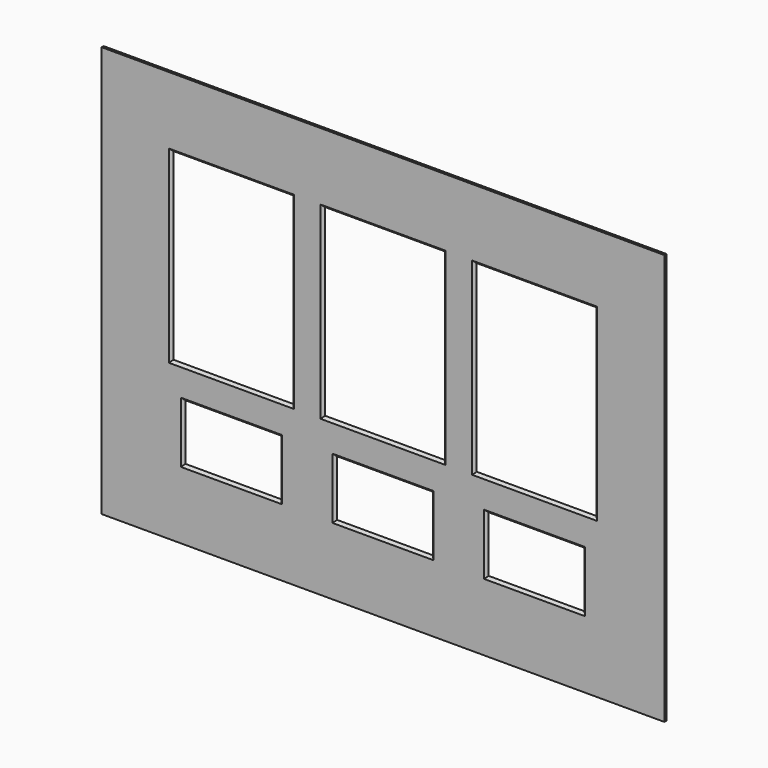
from build123d import *

# Parameters (mm, degrees)
F0_W          = 447.675
F0_H          = 327.025
F0_W_2        = 76.2
F0_H_2        = 44.45
F0_W_3        = 95.25
F0_H_3        = 146.05
F1_DEPTH      = 2
F2_T1_DEPTH   = 95.25
F2_T3_DEPTH   = 146.05
F2_T5_DEPTH   = 95.25
F2_T7_DEPTH   = 95.25
F2_T9_DEPTH   = 76.2
F2_T11_DEPTH  = 44.45
F2_T13_DEPTH  = 76.2
F2_T15_DEPTH  = 76.2
F2_T21_DEPTH  = 151.2756598315
F2_T25_DEPTH  = 100.4756598315
F2_T32_DEPTH  = 100.4756598315
F2_T36_DEPTH  = 151.2756598315
F2_T43_DEPTH  = 151.2756598315
F2_T47_DEPTH  = 100.4756598315
F2_T54_DEPTH  = 151.2756598315
F2_T58_DEPTH  = 100.4756598315
F2_T65_DEPTH  = 151.2756598315
F2_T69_DEPTH  = 100.4756598315
F2_T76_DEPTH  = 151.2756598315
F2_T80_DEPTH  = 100.4756598315
F2_T87_DEPTH  = 100.4756598315
F2_T91_DEPTH  = 151.2756598315
F2_T98_DEPTH  = 151.2756598315
F2_T102_DEPTH = 100.4756598315
F2_T109_DEPTH = 151.2756598315
F2_T113_DEPTH = 100.4756598315
F2_T120_DEPTH = 100.4756598315
F2_T124_DEPTH = 151.2756598315
F2_T131_DEPTH = 151.2756598315
F2_T135_DEPTH = 100.4756598315
F2_T142_DEPTH = 151.2756598315
F2_T146_DEPTH = 100.4756598315
F2_T153_DEPTH = 49.6756598315
F2_T157_DEPTH = 81.4256598315
F2_T164_DEPTH = 81.4256598315
F2_T168_DEPTH = 49.6756598315
F2_T175_DEPTH = 49.6756598315
F2_T179_DEPTH = 81.4256598315
F2_T186_DEPTH = 49.6756598315
F2_T190_DEPTH = 81.4256598315
F2_T197_DEPTH = 81.4256598315
F2_T201_DEPTH = 49.6756598315
F2_T208_DEPTH = 81.4256598315
F2_T212_DEPTH = 49.6756598315
F2_T219_DEPTH = 49.6756598315
F2_T223_DEPTH = 81.4256598315
F2_T230_DEPTH = 81.4256598315
F2_T234_DEPTH = 49.6756598315
F2_T241_DEPTH = 49.6756598315
F2_T245_DEPTH = 81.4256598315
F2_T252_DEPTH = 81.4256598315
F2_T256_DEPTH = 49.6756598315
F2_T263_DEPTH = 81.4256598315
F2_T267_DEPTH = 49.6756598315
F2_T274_DEPTH = 81.4256598315
F2_T278_DEPTH = 49.6756598315


# Not quite as in the source:
# - a fillet or chamfer that OpenCascade refuses, or shapes differently, is made with other operations: its cross-section is extruded or revolved along the edge and cut away or added


with BuildPart() as f1:
    # F0 (on Front) → F1 (new body)
    with BuildSketch(Plane.XZ):
        Rectangle(F0_W, F0_H)
        with Locations((-120.65, -85.725)):
            Rectangle(F0_W_2, F0_H_2, mode=Mode.SUBTRACT)
        with Locations((0, -85.725)):
            Rectangle(F0_W_2, F0_H_2, mode=Mode.SUBTRACT)
        with Locations((120.65, -85.725)):
            Rectangle(F0_W_2, F0_H_2, mode=Mode.SUBTRACT)
        with Locations((-120.65, 34.925)):
            Rectangle(F0_W_3, F0_H_3, mode=Mode.SUBTRACT)
        with Locations((0, 34.925)):
            Rectangle(F0_W_3, F0_H_3, mode=Mode.SUBTRACT)
        with Locations((120.65, 34.925)):
            Rectangle(F0_W_3, F0_H_3, mode=Mode.SUBTRACT)
    extrude(amount=F1_DEPTH)

    # F2: chamfer of 2.032 on 24 edges, made by hand

    # F2_s2 → F2_t1 (cut)
    with BuildSketch(Plane.YZ.offset(-168.275)):
        Polygon((0.032, 107.95), (-2, 109.982), (-2, 107.95), align=None)
        Polygon((0.032, -38.1), (-2, -40.132), (-2, -38.1), align=None)
    extrude(amount=F2_T1_DEPTH, mode=Mode.SUBTRACT)

    # F2_s4 → F2_t3 (cut)
    with BuildSketch(Plane.XY.offset(-38.1)):
        Polygon((-168.275, 0.032), (-170.307, -2), (-168.275, -2), align=None)
        Polygon((-73.025, 0.032), (-70.993, -2), (-73.025, -2), align=None)
        Polygon((-47.625, 0.032), (-49.657, -2), (-47.625, -2), align=None)
        Polygon((47.625, 0.032), (49.657, -2), (47.625, -2), align=None)
        Polygon((73.025, 0.032), (70.993, -2), (73.025, -2), align=None)
        Polygon((168.275, 0.032), (170.307, -2), (168.275, -2), align=None)
    extrude(amount=F2_T3_DEPTH, mode=Mode.SUBTRACT)

    # F2_s6 → F2_t5 (cut)
    with BuildSketch(Plane.YZ.offset(-47.625)):
        Polygon((0.032, 107.95), (-2, 109.982), (-2, 107.95), align=None)
        Polygon((0.032, -38.1), (-2, -40.132), (-2, -38.1), align=None)
    extrude(amount=F2_T5_DEPTH, mode=Mode.SUBTRACT)

    # F2_s8 → F2_t7 (cut)
    with BuildSketch(Plane.YZ.offset(73.025)):
        Polygon((0.032, -38.1), (-2, -40.132), (-2, -38.1), align=None)
        Polygon((0.032, 107.95), (-2, 109.982), (-2, 107.95), align=None)
    extrude(amount=F2_T7_DEPTH, mode=Mode.SUBTRACT)

    # F2_s10 → F2_t9 (cut)
    with BuildSketch(Plane.YZ.offset(82.55)):
        Polygon((0.032, -63.5), (-2, -61.468), (-2, -63.5), align=None)
        Polygon((0.032, -107.95), (-2, -109.982), (-2, -107.95), align=None)
    extrude(amount=F2_T9_DEPTH, mode=Mode.SUBTRACT)

    # F2_s12 → F2_t11 (cut)
    with BuildSketch(Plane.XY.offset(-107.95)):
        Polygon((158.75, 0.032), (160.782, -2), (158.75, -2), align=None)
        Polygon((82.55, 0.032), (80.518, -2), (82.55, -2), align=None)
        Polygon((38.1, 0.032), (40.132, -2), (38.1, -2), align=None)
        Polygon((-38.1, 0.032), (-40.132, -2), (-38.1, -2), align=None)
        Polygon((-82.55, 0.032), (-80.518, -2), (-82.55, -2), align=None)
        Polygon((-158.75, 0.032), (-160.782, -2), (-158.75, -2), align=None)
    extrude(amount=F2_T11_DEPTH, mode=Mode.SUBTRACT)

    # F2_s14 → F2_t13 (cut)
    with BuildSketch(Plane.YZ.offset(-38.1)):
        Polygon((0.032, -63.5), (-2, -61.468), (-2, -63.5), align=None)
        Polygon((0.032, -107.95), (-2, -109.982), (-2, -107.95), align=None)
    extrude(amount=F2_T13_DEPTH, mode=Mode.SUBTRACT)

    # F2_s16 → F2_t15 (cut)
    with BuildSketch(Plane.YZ.offset(-158.75)):
        Polygon((0.032, -107.95), (-2, -109.982), (-2, -107.95), align=None)
        Polygon((0.032, -63.5), (-2, -61.468), (-2, -63.5), align=None)
    extrude(amount=F2_T15_DEPTH, mode=Mode.SUBTRACT)


with BuildPart() as f2_tool19:
    # F2_s20 → F2_t21 (new body)
    with BuildSketch(Plane.XY.offset(-38.1)):
        Polygon((-168.275, 0.032), (-170.307, -2), (-168.275, -2), align=None)
    extrude(amount=F2_T21_DEPTH)

    split(bisect_by=Plane.XY.offset(107.95), keep=Keep.TOP)


with BuildPart() as f2_tool23:
    # F2_s24 → F2_t25 (new body)
    with BuildSketch(Plane.YZ.offset(-173.5006598315)):
        Polygon((0.032, 107.95), (-2, 109.982), (-2, 107.95), align=None)
    extrude(amount=F2_T25_DEPTH)

    split(bisect_by=Plane.YZ.offset(-168.275), keep=Keep.BOTTOM)


with BuildPart() as f2_tool19_1:
    add(f2_tool19.part)

    # F2_t27: intersect F2_tool23
    add(f2_tool23.part, mode=Mode.INTERSECT)


with BuildPart() as f1_1:
    add(f1.part)

    # F2_t17: cut F2_tool19
    add(f2_tool19_1.part, mode=Mode.SUBTRACT)


with BuildPart() as f2_tool30:
    # F2_s31 → F2_t32 (new body)
    with BuildSketch(Plane.YZ.offset(-168.275)):
        Polygon((0.032, 107.95), (-2, 109.982), (-2, 107.95), align=None)
    extrude(amount=F2_T32_DEPTH)

    split(bisect_by=Plane.YZ.offset(-73.025), keep=Keep.TOP)


with BuildPart() as f2_tool34:
    # F2_s35 → F2_t36 (new body)
    with BuildSketch(Plane.XY.offset(113.1756598315)):
        Polygon((-73.025, 0.032), (-70.993, -2), (-73.025, -2), align=None)
    extrude(amount=-F2_T36_DEPTH)

    split(bisect_by=Plane.XY.offset(107.95), keep=Keep.TOP)


with BuildPart() as f2_tool30_1:
    add(f2_tool30.part)

    # F2_t38: intersect F2_tool34
    add(f2_tool34.part, mode=Mode.INTERSECT)


with BuildPart() as f1_2:
    add(f1_1.part)

    # F2_t28: cut F2_tool30
    add(f2_tool30_1.part, mode=Mode.SUBTRACT)


with BuildPart() as f2_tool41:
    # F2_s42 → F2_t43 (new body)
    with BuildSketch(Plane.XY.offset(-43.3256598315)):
        Polygon((-168.275, 0.032), (-170.307, -2), (-168.275, -2), align=None)
    extrude(amount=F2_T43_DEPTH)

    split(bisect_by=Plane.XY.offset(-38.1), keep=Keep.BOTTOM)


with BuildPart() as f2_tool45:
    # F2_s46 → F2_t47 (new body)
    with BuildSketch(Plane.YZ.offset(-73.025)):
        Polygon((0.032, -38.1), (-2, -40.132), (-2, -38.1), align=None)
    extrude(amount=-F2_T47_DEPTH)

    split(bisect_by=Plane.YZ.offset(-168.275), keep=Keep.BOTTOM)


with BuildPart() as f2_tool41_1:
    add(f2_tool41.part)

    # F2_t49: intersect F2_tool45
    add(f2_tool45.part, mode=Mode.INTERSECT)


with BuildPart() as f1_3:
    add(f1_2.part)

    # F2_t39: cut F2_tool41
    add(f2_tool41_1.part, mode=Mode.SUBTRACT)


with BuildPart() as f2_tool52:
    # F2_s53 → F2_t54 (new body)
    with BuildSketch(Plane.XY.offset(107.95)):
        Polygon((-73.025, 0.032), (-70.993, -2), (-73.025, -2), align=None)
    extrude(amount=-F2_T54_DEPTH)

    split(bisect_by=Plane.XY.offset(-38.1), keep=Keep.BOTTOM)


with BuildPart() as f2_tool56:
    # F2_s57 → F2_t58 (new body)
    with BuildSketch(Plane.YZ.offset(-67.7993401685)):
        Polygon((0.032, -38.1), (-2, -40.132), (-2, -38.1), align=None)
    extrude(amount=-F2_T58_DEPTH)

    split(bisect_by=Plane.YZ.offset(-73.025), keep=Keep.TOP)


with BuildPart() as f2_tool52_1:
    add(f2_tool52.part)

    # F2_t60: intersect F2_tool56
    add(f2_tool56.part, mode=Mode.INTERSECT)


with BuildPart() as f1_4:
    add(f1_3.part)

    # F2_t50: cut F2_tool52
    add(f2_tool52_1.part, mode=Mode.SUBTRACT)


with BuildPart() as f2_tool63:
    # F2_s64 → F2_t65 (new body)
    with BuildSketch(Plane.XY.offset(-38.1)):
        Polygon((-47.625, 0.032), (-49.657, -2), (-47.625, -2), align=None)
    extrude(amount=F2_T65_DEPTH)

    split(bisect_by=Plane.XY.offset(107.95), keep=Keep.TOP)


with BuildPart() as f2_tool67:
    # F2_s68 → F2_t69 (new body)
    with BuildSketch(Plane.YZ.offset(-52.8506598315)):
        Polygon((0.032, 107.95), (-2, 109.982), (-2, 107.95), align=None)
    extrude(amount=F2_T69_DEPTH)

    split(bisect_by=Plane.YZ.offset(-47.625), keep=Keep.BOTTOM)


with BuildPart() as f2_tool63_1:
    add(f2_tool63.part)

    # F2_t71: intersect F2_tool67
    add(f2_tool67.part, mode=Mode.INTERSECT)


with BuildPart() as f1_5:
    add(f1_4.part)

    # F2_t61: cut F2_tool63
    add(f2_tool63_1.part, mode=Mode.SUBTRACT)


with BuildPart() as f2_tool74:
    # F2_s75 → F2_t76 (new body)
    with BuildSketch(Plane.XY.offset(113.1756598315)):
        Polygon((47.625, 0.032), (49.657, -2), (47.625, -2), align=None)
    extrude(amount=-F2_T76_DEPTH)

    split(bisect_by=Plane.XY.offset(107.95), keep=Keep.TOP)


with BuildPart() as f2_tool78:
    # F2_s79 → F2_t80 (new body)
    with BuildSketch(Plane.YZ.offset(-47.625)):
        Polygon((0.032, 107.95), (-2, 109.982), (-2, 107.95), align=None)
    extrude(amount=F2_T80_DEPTH)

    split(bisect_by=Plane.YZ.offset(47.625), keep=Keep.TOP)


with BuildPart() as f2_tool74_1:
    add(f2_tool74.part)

    # F2_t82: intersect F2_tool78
    add(f2_tool78.part, mode=Mode.INTERSECT)


with BuildPart() as f1_6:
    add(f1_5.part)

    # F2_t72: cut F2_tool74
    add(f2_tool74_1.part, mode=Mode.SUBTRACT)


with BuildPart() as f2_tool85:
    # F2_s86 → F2_t87 (new body)
    with BuildSketch(Plane.YZ.offset(47.625)):
        Polygon((0.032, -38.1), (-2, -40.132), (-2, -38.1), align=None)
    extrude(amount=-F2_T87_DEPTH)

    split(bisect_by=Plane.YZ.offset(-47.625), keep=Keep.BOTTOM)


with BuildPart() as f2_tool89:
    # F2_s90 → F2_t91 (new body)
    with BuildSketch(Plane.XY.offset(-43.3256598315)):
        Polygon((-47.625, 0.032), (-49.657, -2), (-47.625, -2), align=None)
    extrude(amount=F2_T91_DEPTH)

    split(bisect_by=Plane.XY.offset(-38.1), keep=Keep.BOTTOM)


with BuildPart() as f2_tool85_1:
    add(f2_tool85.part)

    # F2_t93: intersect F2_tool89
    add(f2_tool89.part, mode=Mode.INTERSECT)


with BuildPart() as f1_7:
    add(f1_6.part)

    # F2_t83: cut F2_tool85
    add(f2_tool85_1.part, mode=Mode.SUBTRACT)


with BuildPart() as f2_tool96:
    # F2_s97 → F2_t98 (new body)
    with BuildSketch(Plane.XY.offset(107.95)):
        Polygon((47.625, 0.032), (49.657, -2), (47.625, -2), align=None)
    extrude(amount=-F2_T98_DEPTH)

    split(bisect_by=Plane.XY.offset(-38.1), keep=Keep.BOTTOM)


with BuildPart() as f2_tool100:
    # F2_s101 → F2_t102 (new body)
    with BuildSketch(Plane.YZ.offset(52.8506598315)):
        Polygon((0.032, -38.1), (-2, -40.132), (-2, -38.1), align=None)
    extrude(amount=-F2_T102_DEPTH)

    split(bisect_by=Plane.YZ.offset(47.625), keep=Keep.TOP)


with BuildPart() as f2_tool96_1:
    add(f2_tool96.part)

    # F2_t104: intersect F2_tool100
    add(f2_tool100.part, mode=Mode.INTERSECT)


with BuildPart() as f1_8:
    add(f1_7.part)

    # F2_t94: cut F2_tool96
    add(f2_tool96_1.part, mode=Mode.SUBTRACT)


with BuildPart() as f2_tool107:
    # F2_s108 → F2_t109 (new body)
    with BuildSketch(Plane.XY.offset(107.95)):
        Polygon((168.275, 0.032), (170.307, -2), (168.275, -2), align=None)
    extrude(amount=-F2_T109_DEPTH)

    split(bisect_by=Plane.XY.offset(-38.1), keep=Keep.BOTTOM)


with BuildPart() as f2_tool111:
    # F2_s112 → F2_t113 (new body)
    with BuildSketch(Plane.YZ.offset(173.5006598315)):
        Polygon((0.032, -38.1), (-2, -40.132), (-2, -38.1), align=None)
    extrude(amount=-F2_T113_DEPTH)

    split(bisect_by=Plane.YZ.offset(168.275), keep=Keep.TOP)


with BuildPart() as f2_tool107_1:
    add(f2_tool107.part)

    # F2_t115: intersect F2_tool111
    add(f2_tool111.part, mode=Mode.INTERSECT)


with BuildPart() as f1_9:
    add(f1_8.part)

    # F2_t105: cut F2_tool107
    add(f2_tool107_1.part, mode=Mode.SUBTRACT)


with BuildPart() as f2_tool118:
    # F2_s119 → F2_t120 (new body)
    with BuildSketch(Plane.YZ.offset(168.275)):
        Polygon((0.032, -38.1), (-2, -40.132), (-2, -38.1), align=None)
    extrude(amount=-F2_T120_DEPTH)

    split(bisect_by=Plane.YZ.offset(73.025), keep=Keep.BOTTOM)


with BuildPart() as f2_tool122:
    # F2_s123 → F2_t124 (new body)
    with BuildSketch(Plane.XY.offset(-43.3256598315)):
        Polygon((73.025, 0.032), (70.993, -2), (73.025, -2), align=None)
    extrude(amount=F2_T124_DEPTH)

    split(bisect_by=Plane.XY.offset(-38.1), keep=Keep.BOTTOM)


with BuildPart() as f2_tool118_1:
    add(f2_tool118.part)

    # F2_t126: intersect F2_tool122
    add(f2_tool122.part, mode=Mode.INTERSECT)


with BuildPart() as f1_10:
    add(f1_9.part)

    # F2_t116: cut F2_tool118
    add(f2_tool118_1.part, mode=Mode.SUBTRACT)


with BuildPart() as f2_tool129:
    # F2_s130 → F2_t131 (new body)
    with BuildSketch(Plane.XY.offset(-38.1)):
        Polygon((73.025, 0.032), (70.993, -2), (73.025, -2), align=None)
    extrude(amount=F2_T131_DEPTH)

    split(bisect_by=Plane.XY.offset(107.95), keep=Keep.TOP)


with BuildPart() as f2_tool133:
    # F2_s134 → F2_t135 (new body)
    with BuildSketch(Plane.YZ.offset(67.7993401685)):
        Polygon((0.032, 107.95), (-2, 109.982), (-2, 107.95), align=None)
    extrude(amount=F2_T135_DEPTH)

    split(bisect_by=Plane.YZ.offset(73.025), keep=Keep.BOTTOM)


with BuildPart() as f2_tool129_1:
    add(f2_tool129.part)

    # F2_t137: intersect F2_tool133
    add(f2_tool133.part, mode=Mode.INTERSECT)


with BuildPart() as f1_11:
    add(f1_10.part)

    # F2_t127: cut F2_tool129
    add(f2_tool129_1.part, mode=Mode.SUBTRACT)


with BuildPart() as f2_tool140:
    # F2_s141 → F2_t142 (new body)
    with BuildSketch(Plane.XY.offset(113.1756598315)):
        Polygon((168.275, 0.032), (170.307, -2), (168.275, -2), align=None)
    extrude(amount=-F2_T142_DEPTH)

    split(bisect_by=Plane.XY.offset(107.95), keep=Keep.TOP)


with BuildPart() as f2_tool144:
    # F2_s145 → F2_t146 (new body)
    with BuildSketch(Plane.YZ.offset(73.025)):
        Polygon((0.032, 107.95), (-2, 109.982), (-2, 107.95), align=None)
    extrude(amount=F2_T146_DEPTH)

    split(bisect_by=Plane.YZ.offset(168.275), keep=Keep.TOP)


with BuildPart() as f2_tool140_1:
    add(f2_tool140.part)

    # F2_t148: intersect F2_tool144
    add(f2_tool144.part, mode=Mode.INTERSECT)


with BuildPart() as f1_12:
    add(f1_11.part)

    # F2_t138: cut F2_tool140
    add(f2_tool140_1.part, mode=Mode.SUBTRACT)


with BuildPart() as f2_tool151:
    # F2_s152 → F2_t153 (new body)
    with BuildSketch(Plane.XY.offset(-107.95)):
        Polygon((82.55, 0.032), (80.518, -2), (82.55, -2), align=None)
    extrude(amount=F2_T153_DEPTH)

    split(bisect_by=Plane.XY.offset(-63.5), keep=Keep.TOP)


with BuildPart() as f2_tool155:
    # F2_s156 → F2_t157 (new body)
    with BuildSketch(Plane.YZ.offset(77.3243401685)):
        Polygon((0.032, -63.5), (-2, -61.468), (-2, -63.5), align=None)
    extrude(amount=F2_T157_DEPTH)

    split(bisect_by=Plane.YZ.offset(82.55), keep=Keep.BOTTOM)


with BuildPart() as f2_tool151_1:
    add(f2_tool151.part)

    # F2_t159: intersect F2_tool155
    add(f2_tool155.part, mode=Mode.INTERSECT)


with BuildPart() as f1_13:
    add(f1_12.part)

    # F2_t149: cut F2_tool151
    add(f2_tool151_1.part, mode=Mode.SUBTRACT)


with BuildPart() as f2_tool162:
    # F2_s163 → F2_t164 (new body)
    with BuildSketch(Plane.YZ.offset(82.55)):
        Polygon((0.032, -63.5), (-2, -61.468), (-2, -63.5), align=None)
    extrude(amount=F2_T164_DEPTH)

    split(bisect_by=Plane.YZ.offset(158.75), keep=Keep.TOP)


with BuildPart() as f2_tool166:
    # F2_s167 → F2_t168 (new body)
    with BuildSketch(Plane.XY.offset(-58.2743401685)):
        Polygon((158.75, 0.032), (160.782, -2), (158.75, -2), align=None)
    extrude(amount=-F2_T168_DEPTH)

    split(bisect_by=Plane.XY.offset(-63.5), keep=Keep.TOP)


with BuildPart() as f2_tool162_1:
    add(f2_tool162.part)

    # F2_t170: intersect F2_tool166
    add(f2_tool166.part, mode=Mode.INTERSECT)


with BuildPart() as f1_14:
    add(f1_13.part)

    # F2_t160: cut F2_tool162
    add(f2_tool162_1.part, mode=Mode.SUBTRACT)


with BuildPart() as f2_tool173:
    # F2_s174 → F2_t175 (new body)
    with BuildSketch(Plane.XY.offset(-63.5)):
        Polygon((158.75, 0.032), (160.782, -2), (158.75, -2), align=None)
    extrude(amount=-F2_T175_DEPTH)

    split(bisect_by=Plane.XY.offset(-107.95), keep=Keep.BOTTOM)


with BuildPart() as f2_tool177:
    # F2_s178 → F2_t179 (new body)
    with BuildSketch(Plane.YZ.offset(163.9756598315)):
        Polygon((0.032, -107.95), (-2, -109.982), (-2, -107.95), align=None)
    extrude(amount=-F2_T179_DEPTH)

    split(bisect_by=Plane.YZ.offset(158.75), keep=Keep.TOP)


with BuildPart() as f2_tool173_1:
    add(f2_tool173.part)

    # F2_t181: intersect F2_tool177
    add(f2_tool177.part, mode=Mode.INTERSECT)


with BuildPart() as f1_15:
    add(f1_14.part)

    # F2_t171: cut F2_tool173
    add(f2_tool173_1.part, mode=Mode.SUBTRACT)


with BuildPart() as f2_tool184:
    # F2_s185 → F2_t186 (new body)
    with BuildSketch(Plane.XY.offset(-113.1756598315)):
        Polygon((82.55, 0.032), (80.518, -2), (82.55, -2), align=None)
    extrude(amount=F2_T186_DEPTH)

    split(bisect_by=Plane.XY.offset(-107.95), keep=Keep.BOTTOM)


with BuildPart() as f2_tool188:
    # F2_s189 → F2_t190 (new body)
    with BuildSketch(Plane.YZ.offset(158.75)):
        Polygon((0.032, -107.95), (-2, -109.982), (-2, -107.95), align=None)
    extrude(amount=-F2_T190_DEPTH)

    split(bisect_by=Plane.YZ.offset(82.55), keep=Keep.BOTTOM)


with BuildPart() as f2_tool184_1:
    add(f2_tool184.part)

    # F2_t192: intersect F2_tool188
    add(f2_tool188.part, mode=Mode.INTERSECT)


with BuildPart() as f1_16:
    add(f1_15.part)

    # F2_t182: cut F2_tool184
    add(f2_tool184_1.part, mode=Mode.SUBTRACT)


with BuildPart() as f2_tool195:
    # F2_s196 → F2_t197 (new body)
    with BuildSketch(Plane.YZ.offset(-38.1)):
        Polygon((0.032, -63.5), (-2, -61.468), (-2, -63.5), align=None)
    extrude(amount=F2_T197_DEPTH)

    split(bisect_by=Plane.YZ.offset(38.1), keep=Keep.TOP)


with BuildPart() as f2_tool199:
    # F2_s200 → F2_t201 (new body)
    with BuildSketch(Plane.XY.offset(-58.2743401685)):
        Polygon((38.1, 0.032), (40.132, -2), (38.1, -2), align=None)
    extrude(amount=-F2_T201_DEPTH)

    split(bisect_by=Plane.XY.offset(-63.5), keep=Keep.TOP)


with BuildPart() as f2_tool195_1:
    add(f2_tool195.part)

    # F2_t203: intersect F2_tool199
    add(f2_tool199.part, mode=Mode.INTERSECT)


with BuildPart() as f1_17:
    add(f1_16.part)

    # F2_t193: cut F2_tool195
    add(f2_tool195_1.part, mode=Mode.SUBTRACT)


with BuildPart() as f2_tool206:
    # F2_s207 → F2_t208 (new body)
    with BuildSketch(Plane.YZ.offset(43.3256598315)):
        Polygon((0.032, -107.95), (-2, -109.982), (-2, -107.95), align=None)
    extrude(amount=-F2_T208_DEPTH)

    split(bisect_by=Plane.YZ.offset(38.1), keep=Keep.TOP)


with BuildPart() as f2_tool210:
    # F2_s211 → F2_t212 (new body)
    with BuildSketch(Plane.XY.offset(-63.5)):
        Polygon((38.1, 0.032), (40.132, -2), (38.1, -2), align=None)
    extrude(amount=-F2_T212_DEPTH)

    split(bisect_by=Plane.XY.offset(-107.95), keep=Keep.BOTTOM)


with BuildPart() as f2_tool206_1:
    add(f2_tool206.part)

    # F2_t214: intersect F2_tool210
    add(f2_tool210.part, mode=Mode.INTERSECT)


with BuildPart() as f1_18:
    add(f1_17.part)

    # F2_t204: cut F2_tool206
    add(f2_tool206_1.part, mode=Mode.SUBTRACT)


with BuildPart() as f2_tool217:
    # F2_s218 → F2_t219 (new body)
    with BuildSketch(Plane.XY.offset(-107.95)):
        Polygon((-38.1, 0.032), (-40.132, -2), (-38.1, -2), align=None)
    extrude(amount=F2_T219_DEPTH)

    split(bisect_by=Plane.XY.offset(-63.5), keep=Keep.TOP)


with BuildPart() as f2_tool221:
    # F2_s222 → F2_t223 (new body)
    with BuildSketch(Plane.YZ.offset(-43.3256598315)):
        Polygon((0.032, -63.5), (-2, -61.468), (-2, -63.5), align=None)
    extrude(amount=F2_T223_DEPTH)

    split(bisect_by=Plane.YZ.offset(-38.1), keep=Keep.BOTTOM)


with BuildPart() as f2_tool217_1:
    add(f2_tool217.part)

    # F2_t225: intersect F2_tool221
    add(f2_tool221.part, mode=Mode.INTERSECT)


with BuildPart() as f1_19:
    add(f1_18.part)

    # F2_t215: cut F2_tool217
    add(f2_tool217_1.part, mode=Mode.SUBTRACT)


with BuildPart() as f2_tool228:
    # F2_s229 → F2_t230 (new body)
    with BuildSketch(Plane.YZ.offset(38.1)):
        Polygon((0.032, -107.95), (-2, -109.982), (-2, -107.95), align=None)
    extrude(amount=-F2_T230_DEPTH)

    split(bisect_by=Plane.YZ.offset(-38.1), keep=Keep.BOTTOM)


with BuildPart() as f2_tool232:
    # F2_s233 → F2_t234 (new body)
    with BuildSketch(Plane.XY.offset(-113.1756598315)):
        Polygon((-38.1, 0.032), (-40.132, -2), (-38.1, -2), align=None)
    extrude(amount=F2_T234_DEPTH)

    split(bisect_by=Plane.XY.offset(-107.95), keep=Keep.BOTTOM)


with BuildPart() as f2_tool228_1:
    add(f2_tool228.part)

    # F2_t236: intersect F2_tool232
    add(f2_tool232.part, mode=Mode.INTERSECT)


with BuildPart() as f1_20:
    add(f1_19.part)

    # F2_t226: cut F2_tool228
    add(f2_tool228_1.part, mode=Mode.SUBTRACT)


with BuildPart() as f2_tool239:
    # F2_s240 → F2_t241 (new body)
    with BuildSketch(Plane.XY.offset(-63.5)):
        Polygon((-82.55, 0.032), (-80.518, -2), (-82.55, -2), align=None)
    extrude(amount=-F2_T241_DEPTH)

    split(bisect_by=Plane.XY.offset(-107.95), keep=Keep.BOTTOM)


with BuildPart() as f2_tool243:
    # F2_s244 → F2_t245 (new body)
    with BuildSketch(Plane.YZ.offset(-77.3243401685)):
        Polygon((0.032, -107.95), (-2, -109.982), (-2, -107.95), align=None)
    extrude(amount=-F2_T245_DEPTH)

    split(bisect_by=Plane.YZ.offset(-82.55), keep=Keep.TOP)


with BuildPart() as f2_tool239_1:
    add(f2_tool239.part)

    # F2_t247: intersect F2_tool243
    add(f2_tool243.part, mode=Mode.INTERSECT)


with BuildPart() as f1_21:
    add(f1_20.part)

    # F2_t237: cut F2_tool239
    add(f2_tool239_1.part, mode=Mode.SUBTRACT)


with BuildPart() as f2_tool250:
    # F2_s251 → F2_t252 (new body)
    with BuildSketch(Plane.YZ.offset(-82.55)):
        Polygon((0.032, -107.95), (-2, -109.982), (-2, -107.95), align=None)
    extrude(amount=-F2_T252_DEPTH)

    split(bisect_by=Plane.YZ.offset(-158.75), keep=Keep.BOTTOM)


with BuildPart() as f2_tool254:
    # F2_s255 → F2_t256 (new body)
    with BuildSketch(Plane.XY.offset(-113.1756598315)):
        Polygon((-158.75, 0.032), (-160.782, -2), (-158.75, -2), align=None)
    extrude(amount=F2_T256_DEPTH)

    split(bisect_by=Plane.XY.offset(-107.95), keep=Keep.BOTTOM)


with BuildPart() as f2_tool250_1:
    add(f2_tool250.part)

    # F2_t258: intersect F2_tool254
    add(f2_tool254.part, mode=Mode.INTERSECT)


with BuildPart() as f1_22:
    add(f1_21.part)

    # F2_t248: cut F2_tool250
    add(f2_tool250_1.part, mode=Mode.SUBTRACT)


with BuildPart() as f2_tool261:
    # F2_s262 → F2_t263 (new body)
    with BuildSketch(Plane.YZ.offset(-158.75)):
        Polygon((0.032, -63.5), (-2, -61.468), (-2, -63.5), align=None)
    extrude(amount=F2_T263_DEPTH)

    split(bisect_by=Plane.YZ.offset(-82.55), keep=Keep.TOP)


with BuildPart() as f2_tool265:
    # F2_s266 → F2_t267 (new body)
    with BuildSketch(Plane.XY.offset(-58.2743401685)):
        Polygon((-82.55, 0.032), (-80.518, -2), (-82.55, -2), align=None)
    extrude(amount=-F2_T267_DEPTH)

    split(bisect_by=Plane.XY.offset(-63.5), keep=Keep.TOP)


with BuildPart() as f2_tool261_1:
    add(f2_tool261.part)

    # F2_t269: intersect F2_tool265
    add(f2_tool265.part, mode=Mode.INTERSECT)


with BuildPart() as f1_23:
    add(f1_22.part)

    # F2_t259: cut F2_tool261
    add(f2_tool261_1.part, mode=Mode.SUBTRACT)


with BuildPart() as f2_tool272:
    # F2_s273 → F2_t274 (new body)
    with BuildSketch(Plane.YZ.offset(-163.9756598315)):
        Polygon((0.032, -63.5), (-2, -61.468), (-2, -63.5), align=None)
    extrude(amount=F2_T274_DEPTH)

    split(bisect_by=Plane.YZ.offset(-158.75), keep=Keep.BOTTOM)


with BuildPart() as f2_tool276:
    # F2_s277 → F2_t278 (new body)
    with BuildSketch(Plane.XY.offset(-107.95)):
        Polygon((-158.75, 0.032), (-160.782, -2), (-158.75, -2), align=None)
    extrude(amount=F2_T278_DEPTH)

    split(bisect_by=Plane.XY.offset(-63.5), keep=Keep.TOP)


with BuildPart() as f2_tool272_1:
    add(f2_tool272.part)

    # F2_t280: intersect F2_tool276
    add(f2_tool276.part, mode=Mode.INTERSECT)


with BuildPart() as f1_24:
    add(f1_23.part)

    # F2_t270: cut F2_tool272
    add(f2_tool272_1.part, mode=Mode.SUBTRACT)


solid = f1_24.part
